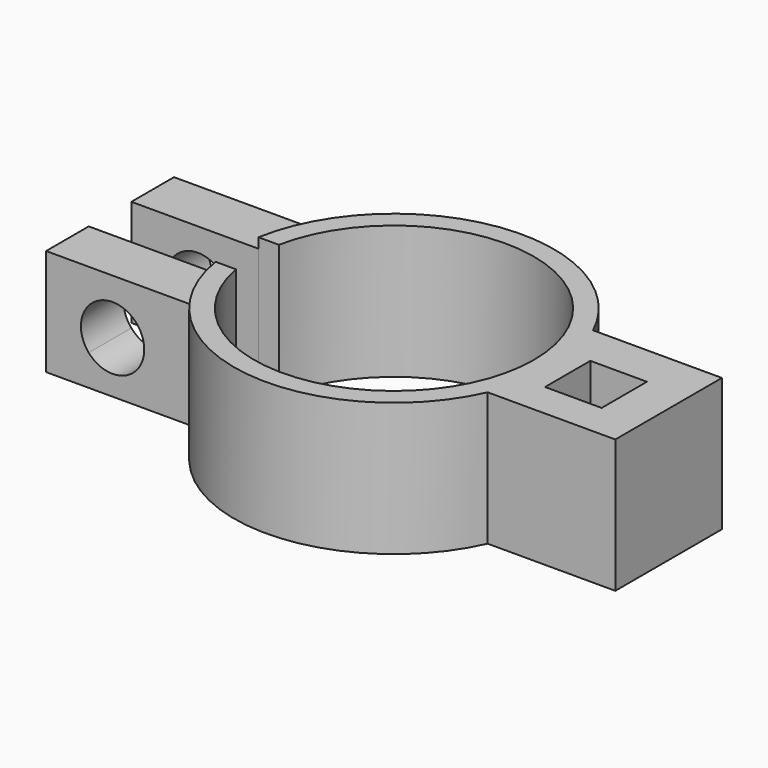
from build123d import *

# Parameters (mm, degrees)
F0_W     = 4.25
F0_H     = 4.25
F1_DEPTH = 5
F3_START = 2
F3_DEPTH = 4
F4_START = -2
F4_DEPTH = 4


# Not quite as in the source:
# - a feature names something its author has since deleted; it is built from what else it names


with BuildPart() as f1:
    # F0 (on Top) → F1 (new body, symmetric)
    with BuildSketch(Plane.XY):
        with BuildLine():
            Line((10.48, -5), (10.48, 5))
            Line((10.48, 5), (0.8137170322, 5))
            ThreePointArc((0.8137170322, 5), (1.6624848855, 2.5140482951), (1.95, -0.0970238614))
            ThreePointArc((1.95, -0.0970238614), (1.6852450978, -2.6038191253), (0.9026629175, -5))
            Line((0.9026629175, -5), (10.48, -5))
        make_face()
        with Locations((5.23, -0.25)):
            Rectangle(F0_W, F0_H, mode=Mode.SUBTRACT)
        with BuildLine():
            ThreePointArc((1.95, -0.0970238614), (1.6624848855, 2.5140482951), (0.8137170322, 5))
            Line((0.8137170322, 5), (0.48, 5))
            Line((0.48, 5), (0.48, -5))
            Line((0.48, -5), (0.9026629175, -5))
            ThreePointArc((0.9026629175, -5), (1.6852450978, -2.6038191253), (1.95, -0.0970238614))
        make_face()
        with BuildLine():
            Line((0.48, 5), (0.8137170322, 5))
            ThreePointArc((0.8137170322, 5), (-11.6370433083, 11.7975670747), (-21.8700390085, 1.9734055232))
            Line((-21.8700390085, 1.9734055232), (-20.3438487537, 1.9734055232))
            ThreePointArc((-20.3438487537, 1.9734055232), (-9.0096663788, 10.3513112192), (0.45, -0.0970238614))
            ThreePointArc((0.45, -0.0970238614), (-9.0810805838, -10.5522232935), (-20.3711800314, -2.0265944768))
            Line((-20.3711800314, -2.0265944768), (-21.89384892, -2.0265944768))
            ThreePointArc((-21.89384892, -2.0265944768), (-11.6020432417, -11.9962323131), (0.9026629175, -5))
            Line((0.9026629175, -5), (0.48, -5))
            Line((0.48, -5), (0.48, 5))
        make_face()
    extrude(amount=F1_DEPTH, both=True)

    # F2 (on Front) → F3 (join)
    with BuildSketch(Plane.XZ.offset(F3_START)):
        with BuildLine():
            Line((-28.1025181167, 1.8032137252), (-31.4321152449, 4.2247389093))
            Line((-31.4321152449, 4.2247389093), (-31.4321152449, -3.7752610907))
            Line((-31.4321152449, -3.7752610907), (-28.2350092218, -1.4500930739))
            ThreePointArc((-28.2350092218, -1.4500930739), (-28.8139991516, 0.2028375775), (-28.1025181167, 1.8032137252))
        make_face()
        with BuildLine():
            Line((-24.4076296068, 1.333455737), (-20.4321152449, 4.2247389093))
            Line((-20.4321152449, 4.2247389093), (-31.4321152449, 4.2247389093))
            Line((-31.4321152449, 4.2247389093), (-28.1025181167, 1.8032137252))
            ThreePointArc((-28.1025181167, 1.8032137252), (-26.1414263845, 2.4622306695), (-24.4076296068, 1.333455737))
        make_face()
        with BuildLine():
            Line((-20.4321152449, -3.7752610907), (-20.4321152449, 0.2247389093))
            Line((-20.4321152449, 0.2247389093), (-20.4321152449, 4.2247389093))
            Line((-20.4321152449, 4.2247389093), (-24.4076296068, 1.333455737))
            ThreePointArc((-24.4076296068, 1.333455737), (-24.1529758873, 0.7431613605), (-24.0659662098, 0.1061956755))
            ThreePointArc((-24.0659662098, 0.1061956755), (-24.128951902, -0.4371410894), (-24.3145681805, -0.9516589557))
            Line((-24.3145681805, -0.9516589557), (-20.4321152449, -3.7752610907))
        make_face()
        with BuildLine():
            Line((-31.4321152449, -3.7752610907), (-20.4321152449, -3.7752610907))
            Line((-20.4321152449, -3.7752610907), (-24.3145681805, -0.9516589557))
            ThreePointArc((-24.3145681805, -0.9516589557), (-26.1414263845, -2.2498393185), (-28.2350092218, -1.4500930739))
            Line((-28.2350092218, -1.4500930739), (-31.4321152449, -3.7752610907))
        make_face()
    extrude(amount=F3_DEPTH)

    # F2 (on Front) → F4 (join)
    with BuildSketch(Plane.XZ.offset(F4_START)):
        with BuildLine():
            Line((-28.1025181167, 1.8032137252), (-31.4321152449, 4.2247389093))
            Line((-31.4321152449, 4.2247389093), (-31.4321152449, -3.7752610907))
            Line((-31.4321152449, -3.7752610907), (-28.2350092218, -1.4500930739))
            ThreePointArc((-28.2350092218, -1.4500930739), (-28.8139991516, 0.2028375775), (-28.1025181167, 1.8032137252))
        make_face()
        with BuildLine():
            Line((-24.4076296068, 1.333455737), (-20.4321152449, 4.2247389093))
            Line((-20.4321152449, 4.2247389093), (-31.4321152449, 4.2247389093))
            Line((-31.4321152449, 4.2247389093), (-28.1025181167, 1.8032137252))
            ThreePointArc((-28.1025181167, 1.8032137252), (-26.1414263845, 2.4622306695), (-24.4076296068, 1.333455737))
        make_face()
        with BuildLine():
            Line((-20.4321152449, -3.7752610907), (-20.4321152449, 0.2247389093))
            Line((-20.4321152449, 0.2247389093), (-20.4321152449, 4.2247389093))
            Line((-20.4321152449, 4.2247389093), (-24.4076296068, 1.333455737))
            ThreePointArc((-24.4076296068, 1.333455737), (-24.1529758873, 0.7431613605), (-24.0659662098, 0.1061956755))
            ThreePointArc((-24.0659662098, 0.1061956755), (-24.128951902, -0.4371410894), (-24.3145681805, -0.9516589557))
            Line((-24.3145681805, -0.9516589557), (-20.4321152449, -3.7752610907))
        make_face()
        with BuildLine():
            Line((-31.4321152449, -3.7752610907), (-20.4321152449, -3.7752610907))
            Line((-20.4321152449, -3.7752610907), (-24.3145681805, -0.9516589557))
            ThreePointArc((-24.3145681805, -0.9516589557), (-26.1414263845, -2.2498393185), (-28.2350092218, -1.4500930739))
            Line((-28.2350092218, -1.4500930739), (-31.4321152449, -3.7752610907))
        make_face()
    extrude(amount=-F4_DEPTH)


solid = f1.part
